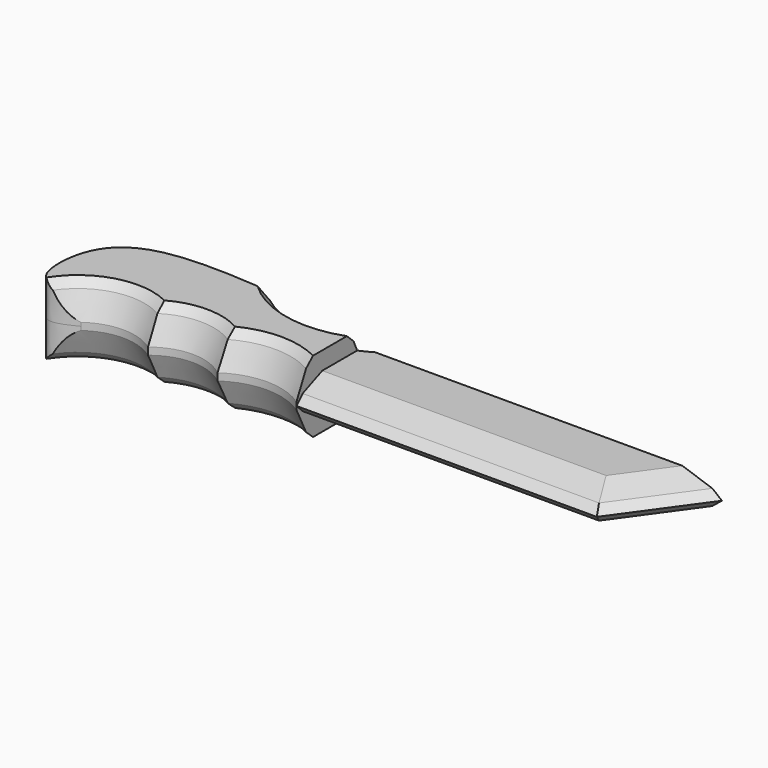
from build123d import *

# Parameters (mm, degrees)
F1_DEPTH      = 6.35
F1_DEPTH_BACK = 6.35
F2_DEPTH      = 12.7
F2_DEPTH_BACK = 12.7
F3_SIZE       = 6.34999
F4_SIZE       = 6.35
F5_T2_ANGLE   = 130.9531767825
F5_T4_ANGLE   = 156.3789559007
F5_T6_ANGLE   = 146.8131509544
F5_T8_ANGLE   = 146.8131509544
F5_T10_ANGLE  = 156.3789559007
F5_T12_ANGLE  = 130.9531767825
F5_T14_ANGLE  = 98.8047724995
F5_T16_ANGLE  = 98.8047724995
F6_SIZE       = 5.08


# Not quite as in the source:
# - a fillet or chamfer that OpenCascade refuses, or shapes differently, is made with other operations: its cross-section is extruded or revolved along the edge and cut away or added
# - a fillet or chamfer is up to 0.001 mm smaller than in the source, because OpenCascade refuses the exact size


with BuildPart() as f1:
    # F0 (on Top) → F1 (new body, two sides)
    with BuildSketch(Plane.XY) as f1_sk:
        Polygon((127.4684071541, 41.98243469), (0, 41.98243469), (0, 12.7772623673), (106.4771935344, 12.7772623673), align=None)
    extrude(amount=F1_DEPTH)
    extrude(f1_sk.sketch, amount=-F1_DEPTH_BACK)

    # F0 (on Top) → F2 (join, two sides)
    with BuildSketch(Plane.XY) as f2_sk:
        with BuildLine():
            Line((0, 12.7772623673), (0, 41.98243469))
            ThreePointArc((0, 41.98243469), (-12.6201109961, 39.2362751187), (-25.2402219921, 41.98243469))
            add(Edge.make_bspline(
                [(-25.2402219921, 41.98243469), (-43.3102802692, 43.6309922068), (-73.0269834828, 46.3420899634), (-90.5393262642, 31.6872008955), (-89.8712560793, 6.151344998), (-80.4582887069, 10.7672416687), (-76.3593539596, 12.7772623673)],
                knots=[0, 0, 0, 0, 0.3656879222, 0.6013837524, 0.8264200944, 1, 1, 1, 1], degree=3))
            ThreePointArc((-76.3593539596, 12.7772623673), (-64.4947532564, 16.6330166618), (-52.6301525533, 12.7772623673))
            ThreePointArc((-52.6301525533, 12.7772623673), (-40.3092205524, 17.1822695756), (-27.9882885516, 12.7772623673))
            ThreePointArc((-27.9882885516, 12.7772623673), (-13.9941442758, 17.1547227044), (0, 12.7772623673))
        make_face()
    extrude(amount=F2_DEPTH)
    extrude(f2_sk.sketch, amount=-F2_DEPTH_BACK)

    # F3 (size 6.35 in the source; OpenCascade refuses exactly that, so slightly less here)
    f3_edges = [f1.edges().sort_by_distance(p)[0] for p in [
        (53.238597, 12.777262, 6.35),
        (116.9728, 27.379849, 6.35),
        (116.9728, 27.379849, -6.35),
        (53.238597, 12.777262, -6.35),
    ]]
    chamfer(f3_edges, length=F3_SIZE)

    # F4
    f4_edges = [f1.edges().sort_by_distance(p)[0] for p in [
        (-40.309221, 17.18227, 12.7),
        (-13.994144, 17.154723, 12.7),
        (-64.494753, 16.633017, 12.7),
        (-13.994144, 17.154723, -12.7),
        (-40.309221, 17.18227, -12.7),
        (-64.494753, 16.633017, -12.7),
        (-12.620111, 39.236275, 12.7),
        (-12.620111, 39.236275, -12.7),
    ]]
    chamfer(f4_edges, length=F4_SIZE)

    # F5: chamfer of 5.08 on 8 edges, made by hand

    # F5_s1 → F5_t2 (revolve, cut)
    with BuildSketch(Plane(origin=(-5.206322323, -11.4118722971, 0), x_dir=(0, 0, 1), z_dir=(-0.415065027, -0.9097917473, 0))):
        Polygon((1.27, 34.2165741448), (9.9421024484, 37.8086765933), (6.35, 34.2165741448), align=None)
    revolve(axis=Axis((-13.9941442758, -7.4026937493, 6.35), (0, 0, -1)), revolution_arc=F5_T2_ANGLE, mode=Mode.SUBTRACT)

    # F5_s3 → F5_t4 (revolve, cut)
    with BuildSketch(Plane(origin=(-2.139660104, -10.2325872802, 0), x_dir=(0, 0, 1), z_dir=(-0.2046758119, -0.9788298177, 0))):
        Polygon((1.27, 58.4285980846), (9.9421024484, 62.020700533), (6.35, 58.4285980846), align=None)
    revolve(axis=Axis((-40.3092205524, -2.2512348183, 6.35), (0, 0, -1)), revolution_arc=F5_T4_ANGLE, mode=Mode.SUBTRACT)

    # F5_s5 → F5_t6 (revolve, cut)
    with BuildSketch(Plane(origin=(-6.2312443492, -20.9110587705, 0), x_dir=(0, 0, 1), z_dir=(-0.2855783849, -0.9583553548, 0))):
        Polygon((1.27, 80.9775575206), (9.9421024484, 84.569659969), (6.35, 80.9775575206), align=None)
    revolve(axis=Axis((-64.4947532564, -3.5492329237, 6.35), (0, 0, -1)), revolution_arc=F5_T6_ANGLE, mode=Mode.SUBTRACT)

    # F5_s7 → F5_t8 (revolve, cut)
    with BuildSketch(Plane(origin=(-6.2312443492, -20.9110587705, 0), x_dir=(0, 0, 1), z_dir=(-0.2855783849, -0.9583553548, 0))):
        Polygon((-1.27, 80.9775575206), (-9.9421024484, 84.569659969), (-6.35, 80.9775575206), align=None)
    revolve(axis=Axis((-64.4947532564, -3.5492329237, -6.35), (0, 0, -1)), revolution_arc=F5_T8_ANGLE, mode=Mode.SUBTRACT)

    # F5_s9 → F5_t10 (revolve, cut)
    with BuildSketch(Plane(origin=(-2.139660104, -10.2325872802, 0), x_dir=(0, 0, 1), z_dir=(-0.2046758119, -0.9788298177, 0))):
        Polygon((-1.27, 58.4285980846), (-9.9421024484, 62.020700533), (-6.35, 58.4285980846), align=None)
    revolve(axis=Axis((-40.3092205524, -2.2512348183, -6.35), (0, 0, -1)), revolution_arc=F5_T10_ANGLE, mode=Mode.SUBTRACT)

    # F5_s11 → F5_t12 (revolve, cut)
    with BuildSketch(Plane(origin=(-5.206322323, -11.4118722971, 0), x_dir=(0, 0, 1), z_dir=(-0.415065027, -0.9097917473, 0))):
        Polygon((-1.27, 34.2165741448), (-9.9421024484, 37.8086765933), (-6.35, 34.2165741448), align=None)
    revolve(axis=Axis((-13.9941442758, -7.4026937493, -6.35), (0, 0, -1)), revolution_arc=F5_T12_ANGLE, mode=Mode.SUBTRACT)

    # F5_s13 → F5_t14 (revolve, cut)
    with BuildSketch(Plane(origin=(29.0494350025, 33.895414243, 0), x_dir=(0, 0, 1), z_dir=(0.6507425946, 0.7592984101, 0))):
        Polygon((9.9421024484, -20.9156595103), (1.27, -24.5077619587), (6.35, -24.5077619587), align=None)
    revolve(axis=Axis((-12.6201109961, 69.6075244238, 6.35), (0, 0, -1)), revolution_arc=F5_T14_ANGLE, mode=Mode.SUBTRACT)

    # F5_s15 → F5_t16 (revolve, cut)
    with BuildSketch(Plane(origin=(29.0494350025, 33.895414243, 0), x_dir=(0, 0, 1), z_dir=(0.6507425946, 0.7592984101, 0))):
        Polygon((-9.9421024484, -20.9156595103), (-1.27, -24.5077619587), (-6.35, -24.5077619587), align=None)
    revolve(axis=Axis((-12.6201109961, 69.6075244238, -6.35), (0, 0, -1)), revolution_arc=F5_T16_ANGLE, mode=Mode.SUBTRACT)

    # F6
    f6_edges = [f1.edges().sort_by_distance(p)[0] for p in [
        (111.434791, 30.554844, -6.35),
        (51.610606, 19.127252, -6.35),
        (111.434791, 30.554844, 6.35),
        (51.610606, 19.127252, 6.35),
    ]]
    chamfer(f6_edges, length=F6_SIZE)


solid = f1.part
